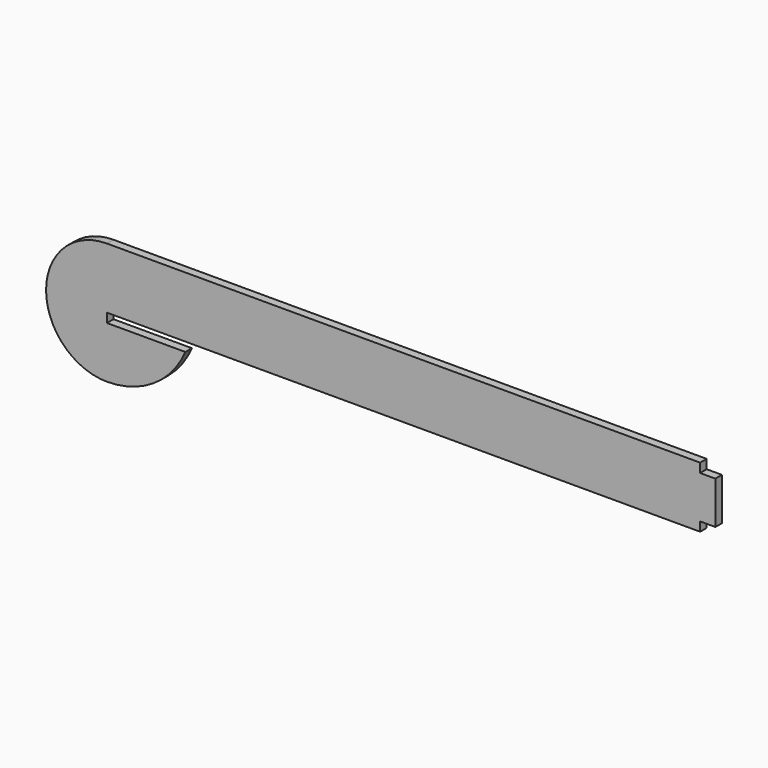
from build123d import *

# Parameters (mm, degrees)
F1_DEPTH = 3.429


# Not quite as in the source:
# - ends of sketch curves that miss each other by under 0.0002 mm in the source are joined


with BuildPart() as f1:
    # F0 (on Front) → F1 (new body)
    with BuildSketch(Plane.XZ):
        with BuildLine():
            Line((412.522035, 410.7526964), (412.522035, 414.5626964))
            Line((412.522035, 414.5626964), (164.872035, 414.5626964))
            ThreePointArc((164.872035, 414.5626964), (139.472035, 389.1626964), (164.872035, 363.7626964))
            ThreePointArc((164.872035, 363.7626964), (184.4881935266, 369.6456603814), (197.6294252739, 385.352696025))
            Line((197.6294252739, 385.352696025), (164.872035, 385.3526964))
            Line((164.872035, 385.3526964), (164.872035, 389.1626964))
            Line((164.872035, 389.1626964), (412.522035, 389.1626964))
            Line((412.522035, 389.1626964), (412.522035, 392.9726964))
            Line((412.522035, 392.9726964), (418.872035, 392.9726964))
            Line((418.872035, 392.9726964), (418.872035, 410.7526964))
            Line((418.872035, 410.7526964), (412.522035, 410.7526964))
        make_face()
    extrude(amount=F1_DEPTH)


solid = f1.part
